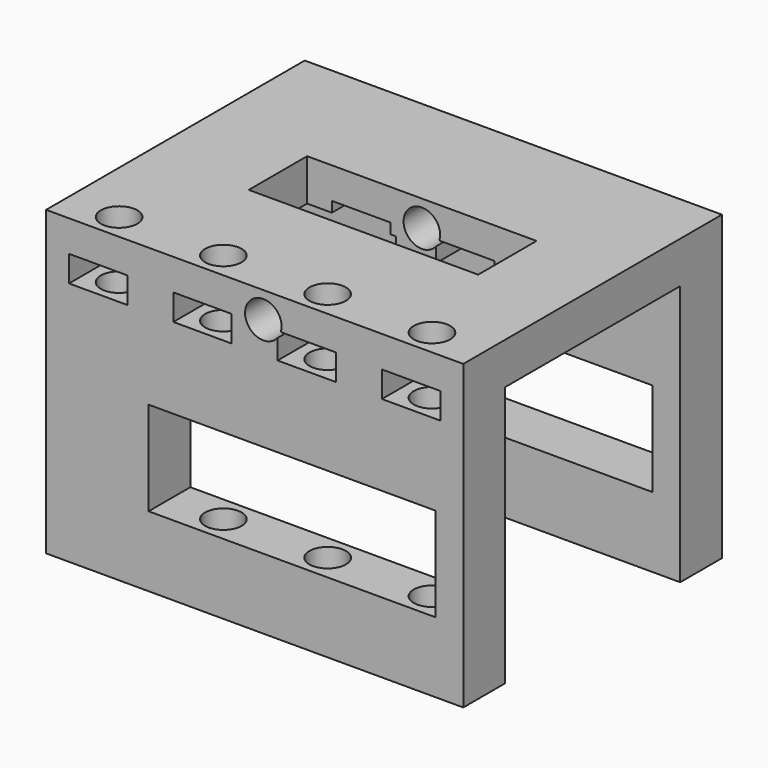
from build123d import *

# Parameters (mm, degrees)
F0_W      = 48.3402396964
F0_H      = 20
F0_W_2    = 22
F0_H_2    = 7
F1_DEPTH  = 4
F3_DEPTH  = 1
F4_R      = 1.75
F5_DEPTH  = 20.001
F6_DEPTH  = 5.5
F7_DEPTH  = 5.5
F8_W      = 21.6701198482
F8_H      = 5
F9_DEPTH  = 25
F10_W     = 21.6701198482
F10_H     = 5
F11_DEPTH = 25
F12_W     = 5
F12_H     = 5
F13_DEPTH = 24
F14_W     = 5
F14_H     = 5
F15_DEPTH = 24
F16_W     = 11
F16_H     = 4.5
F17_DEPTH = 31.001
F19_DEPTH = 29.001
F18_R     = 1.75
F20_DEPTH = 10
F21_W     = 5.6
F21_H     = 2.5
F22_DEPTH = 31.001
F23_DEPTH = 29.001


# Not quite as in the source:
# - a feature names something its author has since deleted; it is built from what else it names


with BuildPart() as f1:
    # F0 (on Top) → F1 (new body)
    with BuildSketch(Plane.XY):
        with Locations((3.7882691845, -5.1383437738)):
            Rectangle(F0_W, F0_H)
        with Locations((3.7882691845, -5.1383437738)):
            Rectangle(F0_W_2, F0_H_2, mode=Mode.SUBTRACT)
    extrude(amount=F1_DEPTH)

    # F2 (on face) → F3 (join)
    with BuildSketch(Plane(origin=(0, 0, 0), x_dir=(1, 0, 0), z_dir=(0, 0, -1))):
        Polygon((6.2882691845, 1.6383437738), (3.7882691845, 1.6383437738), (1.2882691845, 1.6383437738), (1.2882691845, -4.8616562262), (6.2882691845, -4.8616562262), align=None)
        Polygon((1.2882691845, 8.6383437738), (3.7882691845, 8.6383437738), (6.2882691845, 8.6383437738), (6.2882691845, 15.1383437738), (1.2882691845, 15.1383437738), align=None)
    extrude(amount=F3_DEPTH)

    # F4 (on face) → F5 (cut, through all)
    with BuildSketch(Plane.XZ.offset(15.1383437738)):
        with Locations((3.7882691845, 1.5)):
            Circle(F4_R)
    extrude(amount=-F5_DEPTH, mode=Mode.SUBTRACT)

    # F6 (add): a face of the model
    f6_faces = [f1.faces().sort_by_distance(p)[0] for p in [
        (-19.8958693087, -15.1383437738, 2),
    ]]
    extrude(f6_faces, amount=F6_DEPTH)

    # F7 (add): a face of the model
    f7_faces = [f1.faces().sort_by_distance(p)[0] for p in [
        (27.4724076777, 4.8616562262, 2),
    ]]
    extrude(f7_faces, amount=F7_DEPTH)

    # F8 (on face) → F9 (join)
    with BuildSketch(Plane(origin=(0, 0, 0), x_dir=(1, 0, 0), z_dir=(0, 0, -1))):
        with Locations((17.1233291086, -7.8616562262)):
            Rectangle(F8_W, F8_H)
        with Locations((17.1233291086, 18.1383437738)):
            Rectangle(F8_W, F8_H)
    extrude(amount=F9_DEPTH)

    # F10 (on face) → F11 (join)
    with BuildSketch(Plane(origin=(0, 0, 0), x_dir=(1, 0, 0), z_dir=(0, 0, -1))):
        with Locations((-9.5467907396, 18.1383437738)):
            Rectangle(F10_W, F10_H)
        with Locations((-9.5467907396, -7.8616562262)):
            Rectangle(F10_W, F10_H)
    extrude(amount=F11_DEPTH)

    # F12 (on face) → F13 (join)
    with BuildSketch(Plane(origin=(0, 0, -1), x_dir=(1, 0, 0), z_dir=(0, 0, -1))):
        with Locations((3.7882691845, 18.1383437738)):
            Rectangle(F12_W, F12_H)
    extrude(amount=F13_DEPTH)

    # F14 (on face) → F15 (join)
    with BuildSketch(Plane(origin=(0, 0, -1), x_dir=(1, 0, 0), z_dir=(0, 0, -1))):
        with Locations((3.7882691845, -7.8616562262)):
            Rectangle(F14_W, F14_H)
    extrude(amount=F15_DEPTH)

    # F16 (on face) → F17 (cut, through all)
    with BuildSketch(Plane.XZ.offset(20.6383437738)):
        with Locations((9.2882691845, -16)):
            Rectangle(F16_W, F16_H)
        Polygon((3.7882691845, -18.25), (3.7882691845, -13.75), (14.7882691845, -13.75), (14.7882691845, -9.25), (-7.2117308155, -9.25), (-7.2117308155, -18.25), align=None)
        Polygon((14.7882691845, -9.25), (14.7882691845, -13.75), (14.7882691845, -18.25), (20.2882691845, -18.25), (20.2882691845, -9.25), align=None)
    extrude(amount=-F17_DEPTH, mode=Mode.SUBTRACT)

    # F18 (on face) → F19 (cut, through all)
    with BuildSketch(Plane.XY.offset(4)):
        Polygon((-20.3818506637, -20.6383437738), (-17.0416109673, -20.6383437738), (-17.0416109673, -5.1383437738), (-17.0416109673, 10.3616562262), (-20.3818506637, 10.3616562262), align=None)
    extrude(amount=-F19_DEPTH, mode=Mode.SUBTRACT)

    # F18 (on face) → F20 (cut)
    with BuildSketch(Plane.XY.offset(4)):
        with Locations((-12.0416109673, -18.1383437738)):
            Circle(F18_R)
    extrude(amount=-F20_DEPTH, mode=Mode.SUBTRACT)

    # F21 (on face) → F22 (cut, through all)
    with BuildSketch(Plane.XZ.offset(20.6383437738)):
        Polygon((-12.0416109673, 1), (-14.8416109673, 1), (-14.8416109673, -1.5), (-9.2416109673, -1.5), (-9.2416109673, 1), align=None)
        Polygon((27.9583890327, 4), (22.9583890327, 4), (22.9583890327, 1), (22.9583890327, -25), (27.9583890327, -25), align=None)
        with Locations((-2.0416109673, -0.25)):
            Rectangle(F21_W, F21_H)
        with BuildLine():
            Line((5.1583890327, 0.4112982035), (5.1583890327, -1.5))
            Line((5.1583890327, -1.5), (10.7583890327, -1.5))
            Line((10.7583890327, -1.5), (10.7583890327, 1))
            Line((10.7583890327, 1), (5.4653201677, 1))
            ThreePointArc((5.4653201677, 1), (5.3400278546, 0.6909604275), (5.1583890327, 0.4112982035))
        make_face()
        Polygon((20.7583890327, -1.5), (20.7583890327, 1), (17.9583890327, 1), (15.1583890327, 1), (15.1583890327, -1.5), align=None)
    extrude(amount=-F22_DEPTH, mode=Mode.SUBTRACT)

    # F18 (on face) → F23 (cut, through all)
    with BuildSketch(Plane.XY.offset(4)):
        Polygon((-17.0416109673, -20.6383437738), (-17.0416109673, -5.1383437738), (-17.0416109673, 10.3616562262), (-20.3818506637, 10.3616562262), (-20.3818506637, -20.6383437738), align=None)
        with Locations((-12.0416109673, -18.1383437738)):
            Circle(F18_R)
        with BuildLine():
            ThreePointArc((19.7083890327, -18.1383437738), (17.9583890327, -16.3883437738), (16.2083890327, -18.1383437738))
            ThreePointArc((16.2083890327, -18.1383437738), (17.9583890327, -19.8883437738), (19.7083890327, -18.1383437738))
        make_face()
        with BuildLine():
            ThreePointArc((9.7083890327, -18.1383437738), (7.9583890327, -16.3883437738), (6.2083890327, -18.1383437738))
            Line((6.2083890327, -18.1383437738), (7.9583890327, -18.1383437738))
            Line((7.9583890327, -18.1383437738), (9.7083890327, -18.1383437738))
        make_face()
        with BuildLine():
            Line((7.9583890327, -18.1383437738), (6.2083890327, -18.1383437738))
            ThreePointArc((6.2083890327, -18.1383437738), (7.9583890327, -19.8883437738), (9.7083890327, -18.1383437738))
            Line((9.7083890327, -18.1383437738), (7.9583890327, -18.1383437738))
        make_face()
        with BuildLine():
            ThreePointArc((-0.2916109673, -18.1383437738), (-2.0416109673, -16.3883437738), (-3.7916109673, -18.1383437738))
            Line((-3.7916109673, -18.1383437738), (-2.0416109673, -18.1383437738))
            Line((-2.0416109673, -18.1383437738), (-0.2916109673, -18.1383437738))
        make_face()
        with BuildLine():
            Line((-2.0416109673, -18.1383437738), (-3.7916109673, -18.1383437738))
            ThreePointArc((-3.7916109673, -18.1383437738), (-2.0416109673, -19.8883437738), (-0.2916109673, -18.1383437738))
            Line((-0.2916109673, -18.1383437738), (-2.0416109673, -18.1383437738))
        make_face()
    extrude(amount=-F23_DEPTH, mode=Mode.SUBTRACT)


solid = f1.part
